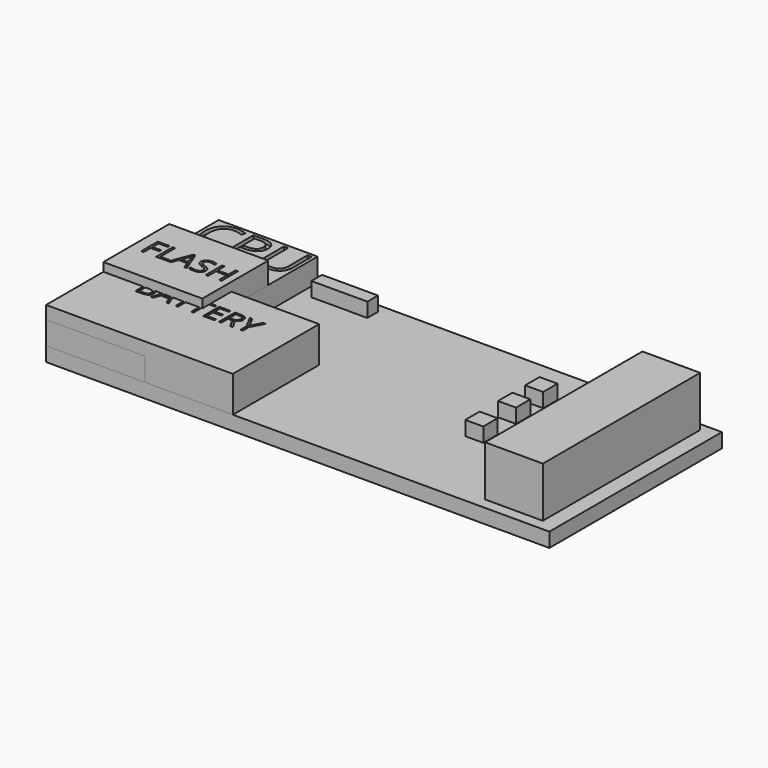
from build123d import *

# Parameters (mm, degrees)
F1_W          = 5.4390531281
F1_H          = 5.4520857245
F2_DEPTH      = 2.54
F1_W_2        = 2.3118479828
F1_H_2        = 5.9173218804
F1_W_3        = 3.175
F1_H_3        = 3.175
F1_W_4        = 9.8876314243
F1_H_4        = 2.3438557982
F0_W          = 88.9
F0_H          = 38.1
F3_DEPTH      = 2.54
F4_W          = 32.9911390568
F4_H          = 19.05
F5_DEPTH      = 6.35
F6_TEXT_SIZE  = 5.0115502543
F7_DEPTH      = 0.254
F8_W          = 10.2006465895
F8_H          = 34.7317848355
F9_DEPTH      = 8.89
F10_W         = 17.4822861577
F10_H         = 38.1
F11_DEPTH     = 4.064
F12_TEXT_SIZE = 9.0347732081
F13_DEPTH     = 0.635
F14_W         = 17.4822861577
F14_H         = 14.53769207
F15_DEPTH     = 3.81
F16_TEXT_SIZE = 5.1335638596
F17_DEPTH     = 1.27


# Not quite as in the source:
# - Text() gives the source's letters only with a copy of the font that has no kerning and outlines rounded to 1/6400 em; it was checked with that copy


with BuildPart() as f2:
    # F1 (on face) → F2 (new body)
    with BuildSketch(Plane.XY):
        with Locations((-71.2464059123, -39.8216265268)):
            Rectangle(F1_W, F1_H)
    extrude(amount=F2_DEPTH)


with BuildPart() as f2b:
    # F1 (on face) → F2, piece 2 (new body)
    with BuildSketch(Plane.XY):
        with Locations((-63.8960185141, -53.0489546422)):
            Rectangle(F1_W_2, F1_H_2)
    extrude(amount=F2_DEPTH)


with BuildPart() as f2c:
    # F1 (on face) → F2, piece 3 (new body)
    with BuildSketch(Plane.XY):
        with Locations((-20.9667075921, -35.2881999017)):
            Rectangle(F1_W_3, F1_H_3)
    extrude(amount=F2_DEPTH)


with BuildPart() as f2d:
    # F1 (on face) → F2, piece 4 (new body)
    with BuildSketch(Plane.XY):
        with Locations((-14.3407390503, -35.2881999017)):
            Rectangle(F1_W_3, F1_H_3)
    extrude(amount=F2_DEPTH)


with BuildPart() as f2e:
    # F1 (on face) → F2, piece 5 (new body)
    with BuildSketch(Plane.XY):
        with Locations((-20.9667075921, -41.2729425234)):
            Rectangle(F1_W_3, F1_H_3)
    extrude(amount=F2_DEPTH)


with BuildPart() as f2f:
    # F1 (on face) → F2, piece 6 (new body)
    with BuildSketch(Plane.XY):
        with Locations((-14.3407390503, -41.2729425234)):
            Rectangle(F1_W_3, F1_H_3)
    extrude(amount=F2_DEPTH)


with BuildPart() as f2g:
    # F1 (on face) → F2, piece 7 (new body)
    with BuildSketch(Plane.XY):
        with Locations((-20.9667075921, -48.502793702)):
            Rectangle(F1_W_3, F1_H_3)
    extrude(amount=F2_DEPTH)


with BuildPart() as f2h:
    # F1 (on face) → F2, piece 8 (new body)
    with BuildSketch(Plane.XY):
        with Locations((-14.3407390503, -48.502793702)):
            Rectangle(F1_W_3, F1_H_3)
    extrude(amount=F2_DEPTH)


with BuildPart() as f2i:
    # F1 (on face) → F2, piece 9 (new body)
    with BuildSketch(Plane.XY):
        with Locations((-60.1081267933, -29.7783128917)):
            Rectangle(F1_W_4, F1_H_4)
    extrude(amount=F2_DEPTH)


with BuildPart() as f3:
    # F0 (on Top) → F3 (new body)
    with BuildSketch(Plane.XY):
        with Locations((-40.1366704608, -46.0612718016)):
            Rectangle(F0_W, F0_H)
    extrude(amount=-F3_DEPTH)


with BuildPart() as f5:
    # F4 (on face) → F5 (new body)
    with BuildSketch(Plane.XY):
        with Locations((-68.0911009324, -55.5862718016)):
            Rectangle(F4_W, F4_H)
    extrude(amount=F5_DEPTH)

    # F6 (on face) → F7 (cut)
    with BuildSketch(Plane.XY.offset(6.35)):
        with Locations((-78.0573636293, -54.1880838573)):
            Text('BATTERY', F6_TEXT_SIZE, font='Open Sans', text_align=(TextAlign.LEFT, TextAlign.BOTTOM))
    extrude(amount=-F7_DEPTH, mode=Mode.SUBTRACT)


with BuildPart() as f9:
    # F8 (on face) → F9 (new body)
    with BuildSketch(Plane.XY):
        with Locations((-3.5195067176, -45.7659913227)):
            Rectangle(F8_W, F8_H)
    extrude(amount=F9_DEPTH)


with BuildPart() as f11:
    # F10 (on face) → F11 (new body)
    with BuildSketch(Plane.XY):
        with Locations((-75.845527382, -46.0612718016)):
            Rectangle(F10_W, F10_H)
    extrude(amount=F11_DEPTH)

    # F12 (on face) → F13 (cut)
    with BuildSketch(Plane.XY.offset(4.064)):
        with Locations((-84.5866704608, -34.0158467436)):
            Text('CPU', F12_TEXT_SIZE, font='Open Sans', text_align=(TextAlign.LEFT, TextAlign.BOTTOM))
    extrude(amount=-F13_DEPTH, mode=Mode.SUBTRACT)


with BuildPart() as f15:
    # F14 (on face) → F15 (new body)
    with BuildSketch(Plane.XY.offset(4.064)):
        with Locations((-75.845527382, -45.1850071549)):
            Rectangle(F14_W, F14_H)
    extrude(amount=F15_DEPTH)

    # F16 (on face) → F17 (cut)
    with BuildSketch(Plane.XY.offset(7.874)):
        with Locations((-83.0357298255, -46.6768629849)):
            Text('FLASH', F16_TEXT_SIZE, font='Open Sans', text_align=(TextAlign.LEFT, TextAlign.BOTTOM))
    extrude(amount=-F17_DEPTH, mode=Mode.SUBTRACT)


solid = Compound([f2.part, f2b.part, f2c.part, f2d.part, f2e.part, f2f.part, f2g.part, f2h.part, f2i.part, f3.part, f5.part, f9.part, f11.part, f15.part])
